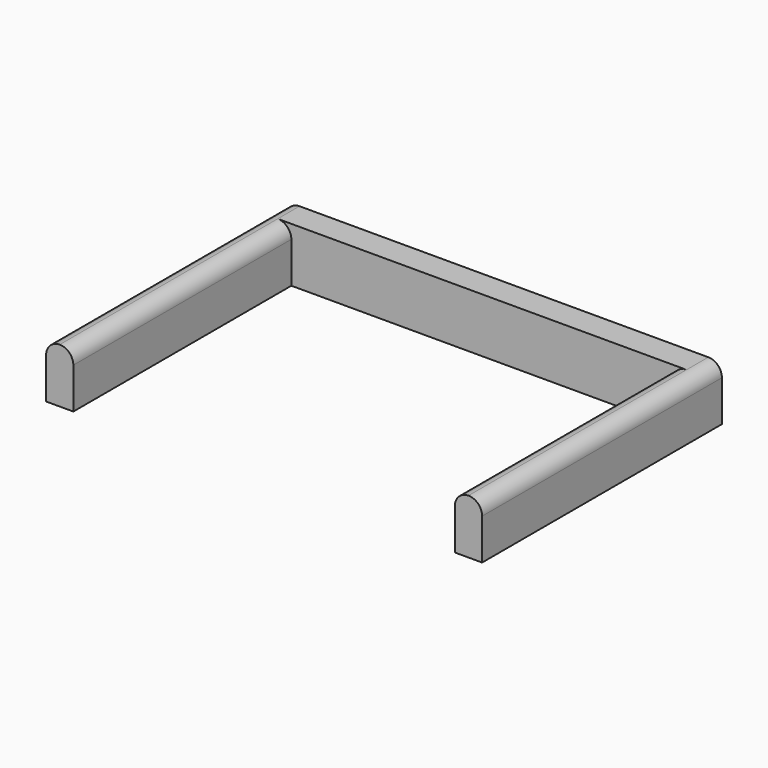
from build123d import *

# Parameters (mm, degrees)
F1_DEPTH = 10
F2_R     = 2.49999


# Not quite as in the source:
# - a fillet or chamfer is up to 0.001 mm smaller than in the source, because OpenCascade refuses the exact size


with BuildPart() as f1:
    # F0 (on Top) → F1 (new body)
    with BuildSketch(Plane.XY):
        Polygon((-44.6886586582, 25.7738458982), (-44.6886586582, -29.2261541018), (-39.6886586582, -29.2261541018), (-39.6886586582, 20.7738458982), (30.3113413418, 20.7738458982), (30.3113413418, -29.2261541018), (35.3113413418, -29.2261541018), (35.3113413418, 25.7738458982), align=None)
    extrude(amount=F1_DEPTH)

    # F2 (radius 2.5 in the source; OpenCascade refuses exactly that, so slightly less here)
    f2_edges = [f1.edges().sort_by_distance(p)[0] for p in [
        (-44.688659, -1.726154, 10),
        (-39.688659, -4.226154, 10),
        (30.311341, -4.226154, 10),
        (35.311341, -1.726154, 10),
    ]]
    fillet(f2_edges, radius=F2_R)


solid = f1.part
